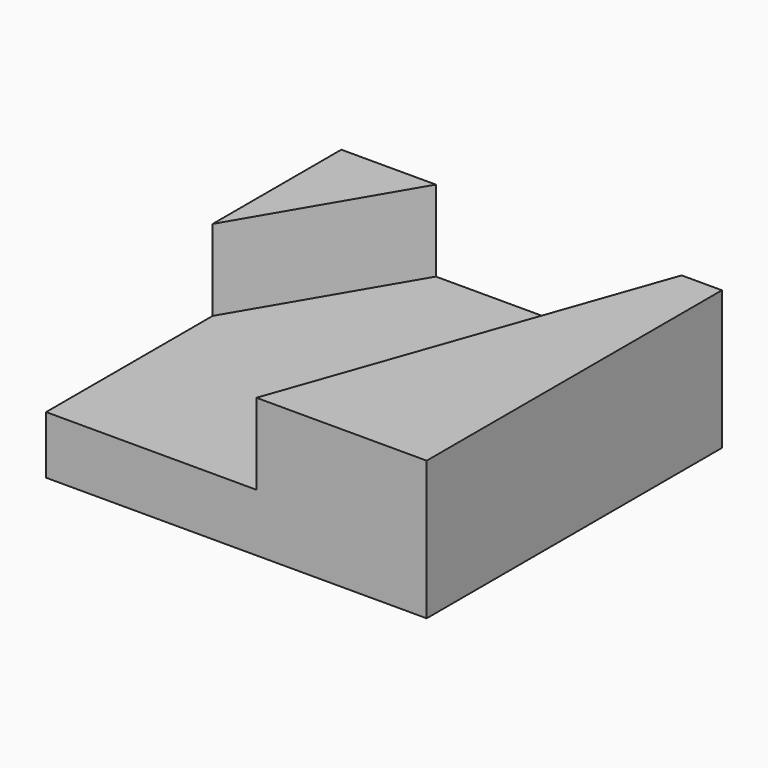
from build123d import *

# Parameters (mm, degrees)
F0_W      = 50.8
F0_H      = 30.48
F1_DEPTH  = 25.4
F2_DEPTH  = 55.626
F3_DEPTH  = 32.766
F6_DEPTH  = 25.4
F7_DEPTH  = 25.4
F9_DEPTH  = 25.4
F10_DEPTH = 7.62


with BuildPart() as f1:
    # F0 (on Front) → F1 (new body)
    with BuildSketch(Plane.XZ):
        with Locations((-32.1067409651, 15.24)):
            Rectangle(F0_W, F0_H)
    extrude(amount=F1_DEPTH)

    # F2 (add): a face of the model
    f2_faces = [f1.faces().sort_by_distance(p)[0] for p in [
        (-32.1067409651, 0, 15.24),
    ]]
    extrude(f2_faces, amount=F2_DEPTH)

    # F3 (add): a face of the model
    f3_faces = [f1.faces().sort_by_distance(p)[0] for p in [
        (-6.7067409651, 15.113, 15.24),
    ]]
    extrude(f3_faces, amount=F3_DEPTH)

    # F4 (on face) → F6 (cut)
    with BuildSketch(Plane.XY.offset(30.48)):
        Polygon((-11.3192433491, -25.4), (17.2114539891, 55.626), (-57.5067409651, 55.626), (-57.5067409651, -25.4), align=None)
    extrude(amount=-F6_DEPTH, mode=Mode.SUBTRACT)

    # F5 (on face) → F7 (cut)
    with BuildSketch(Plane.XY.offset(30.48)):
        Polygon((-57.5067409651, -25.4), (-11.3192433491, -25.4), (17.2114539891, 55.626), (-43.2823600247, 55.626), (-57.5067409651, 55.626), align=None)
    extrude(amount=-F7_DEPTH, mode=Mode.SUBTRACT)

    # F8 (on face) → F9 (join)
    with BuildSketch(Plane.XY.offset(5.08)):
        Polygon((-57.5067409651, 20.3126166016), (-36.7487818003, 55.626), (-57.5067409651, 55.626), align=None)
    extrude(amount=F9_DEPTH)

    # F10 (add): a face of the model
    f10_faces = [f1.faces().sort_by_distance(p)[0] for p in [
        (-24.788870281, 16.2328343869, 5.08),
    ]]
    extrude(f10_faces, amount=F10_DEPTH)


solid = f1.part
